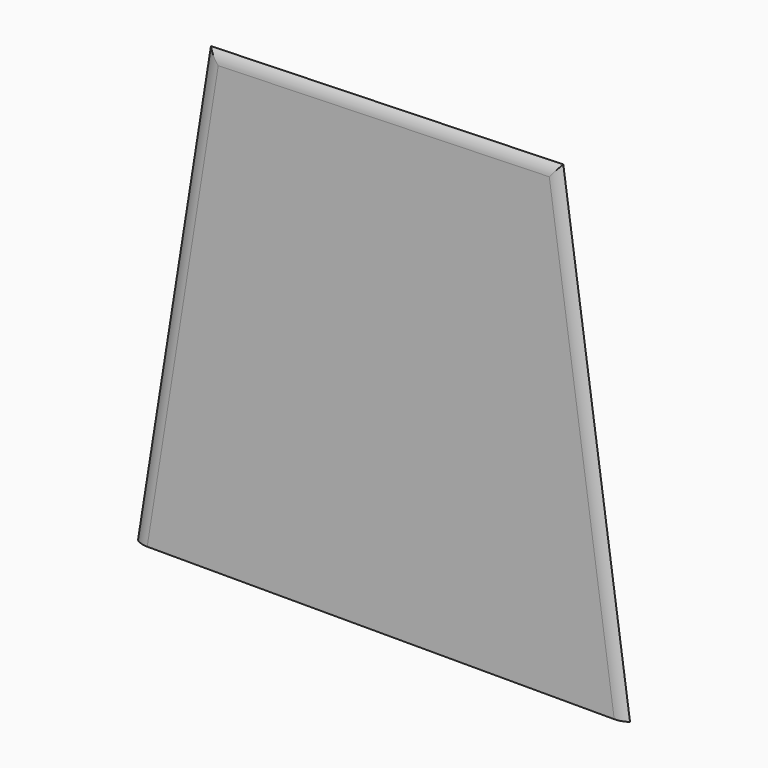
from build123d import *

# Parameters (mm, degrees)
F1_DEPTH    = 1
F2_T1_DEPTH = 127.5241695926
F2_T3_DEPTH = 129.7959329915
F2_T5_DEPTH = 100.4028232355


# Not quite as in the source:
# - a fillet or chamfer that OpenCascade refuses, or shapes differently, is made with other operations: its cross-section is extruded or revolved along the edge and cut away or added


with BuildPart() as f1:
    # F0 (on Front) → F1 (new body)
    with BuildSketch(Plane.XZ):
        Polygon((43.9455360174, 64.9080649018), (-41.4199344814, 62.3824633658), (-59.099175036, -48.7441904843), (60.1094178855, -48.7441904843), align=None)
    extrude(amount=F1_DEPTH)

    # F2: fillet of radius 5 on 3 edges, made by hand

    # F2_s2 → F2_t1 (cut)
    with BuildSketch(Plane(origin=(9.8354016997, 0, 61.8225243777), x_dir=(0, 1, 0), z_dir=(-0.1571150502, 0, -0.9875803061))):
        with BuildLine():
            ThreePointArc((0, -50.7067354373), (-0.7434164903, -49.2878742674), (-1, -47.7067354373))
            Line((-1, -47.7067354373), (-1, -50.7067354373))
            Line((-1, -50.7067354373), (0, -50.7067354373))
        make_face()
    extrude(amount=F2_T1_DEPTH, mode=Mode.SUBTRACT)

    # F2_s4 → F2_t3 (cut)
    with BuildSketch(Plane(origin=(9.0428428438, 0, -63.5824669276), x_dir=(0, 1, 0), z_dir=(-0.140805353, 0, 0.9900372986))):
        with BuildLine():
            ThreePointArc((0, -52.6471227542), (-0.7434164903, -51.2282615843), (-1, -49.6471227542))
            Line((-1, -49.6471227542), (-1, -52.6471227542))
            Line((-1, -52.6471227542), (0, -52.6471227542))
        make_face()
    extrude(amount=F2_T3_DEPTH, mode=Mode.SUBTRACT)

    # F2_s6 → F2_t5 (cut)
    with BuildSketch(Plane(origin=(53.3224974993, 0, 1.5775861224), x_dir=(0, 1, 0), z_dir=(-0.9995626288, 0, -0.0295728108))):
        with BuildLine():
            ThreePointArc((0, -63.5800829589), (-0.7434164903, -62.161221789), (-1, -60.5800829589))
            Line((-1, -60.5800829589), (-1, -63.5800829589))
            Line((-1, -63.5800829589), (0, -63.5800829589))
        make_face()
    extrude(amount=F2_T5_DEPTH, mode=Mode.SUBTRACT)


solid = f1.part
